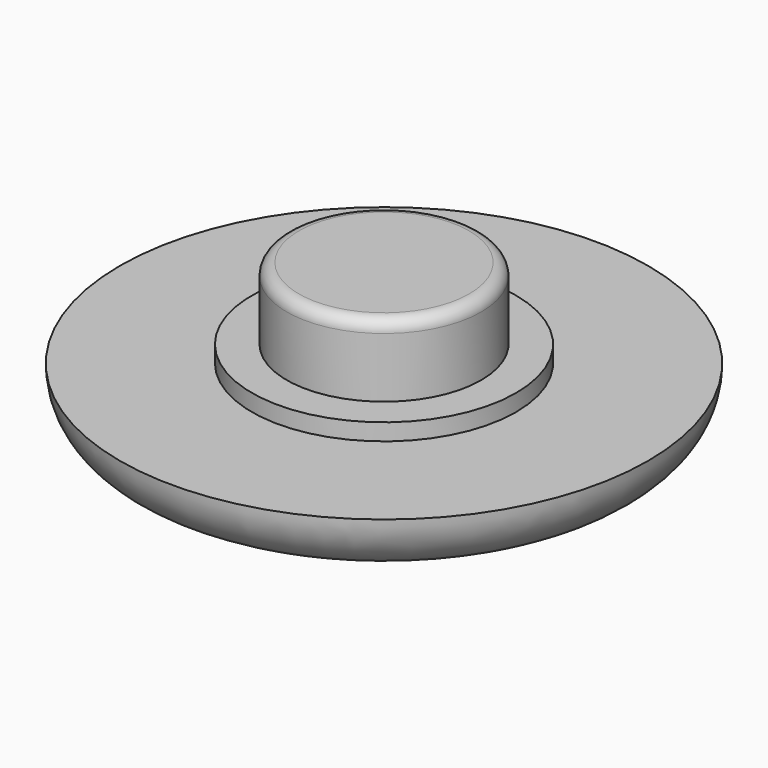
from build123d import *

# Parameters (mm, degrees)
F0_R     = 11
F0_R_2   = 5.5
F1_DEPTH = 2.5
F0_R_3   = 4.05
F2_DEPTH = 3.2
F3_DEPTH = 6.2
F4_R     = 2.49999
F5_R     = 0.5


# Not quite as in the source:
# - a fillet or chamfer is up to 0.001 mm smaller than in the source, because OpenCascade refuses the exact size


with BuildPart() as f1:
    # F0 (on Top) → F1 (new body)
    with BuildSketch(Plane.XY):
        Circle(F0_R)
        Circle(F0_R_2, mode=Mode.SUBTRACT)
    extrude(amount=F1_DEPTH)

    # F0 (on Top) → F2 (join)
    with BuildSketch(Plane.XY):
        Circle(F0_R_2)
        Circle(F0_R_3, mode=Mode.SUBTRACT)
    extrude(amount=F2_DEPTH)

    # F0 (on Top) → F3 (join)
    with BuildSketch(Plane.XY):
        Circle(F0_R_3)
    extrude(amount=F3_DEPTH)

    # F4 (radius 2.5 in the source; OpenCascade refuses exactly that, so slightly less here)
    f4_edges = [f1.edges().sort_by_distance(p)[0] for p in [
        (-11, 0, 0),
    ]]
    fillet(f4_edges, radius=F4_R)

    # F5
    f5_edges = [f1.edges().sort_by_distance(p)[0] for p in [
        (-4.05, 0, 6.2),
    ]]
    fillet(f5_edges, radius=F5_R)


solid = f1.part
